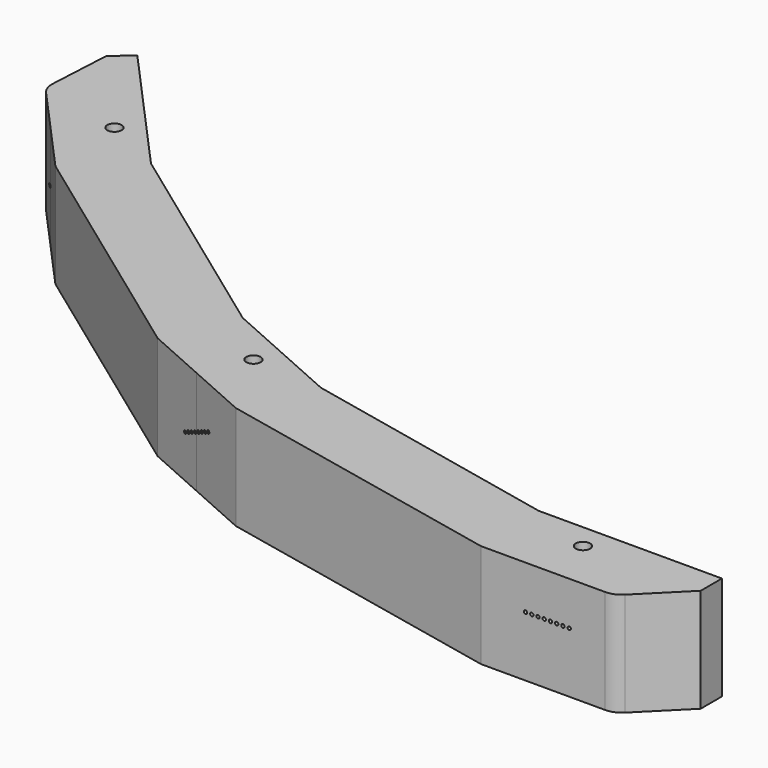
from build123d import *

# Parameters (mm, degrees)
F1_DEPTH        = 25
F2_W            = 17
F2_H            = 14
F3_DEPTH        = 10
F4_W            = 12
F4_H            = 12
F5_DEPTH        = 10
F7_D            = 0.8
F7_CSINK_D      = 0.866
F7_CSINK_ANGLE  = 60
F9_D            = 0.8
F9_CSINK_D      = 0.866
F9_CSINK_ANGLE  = 60
F10_W           = 17
F10_H           = 14
F11_DEPTH       = 10
F13_D           = 0.8
F13_CSINK_D     = 0.866
F13_CSINK_ANGLE = 60
F15_DEPTH       = 1
F17_DEPTH       = 1
F19_DEPTH       = 1
F21_D           = 3.4544
F21_DEPTH       = 14.38125
F21_TIP         = 1.0378064612
F23_D           = 4.2
F23_DEPTH       = 10
F23_TIP         = 1.2618073
F24_R           = 0.5
F25_R           = 0.5
F26_R           = 0.5
F28_D           = 4.2
F28_DEPTH       = 10
F28_TIP         = 1.2618073
F30_D           = 4.2
F30_DEPTH       = 10
F30_TIP         = 1.2618073
F32_D           = 3.02
F32_DEPTH       = 6
F32_TIP         = 0.9072995347
F34_D           = 3.02
F34_DEPTH       = 6
F34_TIP         = 0.9072995347


# Not quite as in the source:
# - a feature names something its author has since deleted; it is built from what else it names


with BuildPart() as f1:
    # F0 (on Top) → F1 (new body)
    with BuildSketch(Plane.XY):
        with BuildLine():
            Line((-195.1064812103, -156.9314377097), (-185.7862063693, -167.2826515897))
            Line((-185.7862063693, -167.2826515897), (-175.0801166676, -179.1729687974))
            Line((-175.0801166676, -179.1729687974), (-116.3008880912, -221.8785781214))
            Line((-116.3008880912, -221.8785781214), (-101.6841607689, -228.3863644107))
            Line((-101.6841607689, -228.3863644107), (-87.0674334467, -234.8941506999))
            Line((-87.0674334467, -234.8941506999), (-16, -250))
            Line((-16, -250), (0, -250))
            Line((0, -250), (13.9289321881, -250))
            ThreePointArc((13.9289321881, -250), (15.84234935, -249.6193976626), (17.4644660941, -248.5355339059))
            Line((17.4644660941, -248.5355339059), (27.610408524, -238.389591476))
            Line((27.610408524, -238.389591476), (27.610408524, -232))
            Line((27.610408524, -232), (-0.4985836237, -232))
            Line((-0.4985836237, -232), (-16.4985836237, -232))
            Line((-16.4985836237, -232), (-79.7461738713, -218.4503324623))
            Line((-79.7461738713, -218.4503324623), (-94.3629011936, -211.9425461731))
            Line((-94.3629011936, -211.9425461731), (-108.9796285159, -205.4347598839))
            Line((-108.9796285159, -205.4347598839), (-161.703509809, -167.1286178829))
            Line((-161.703509809, -167.1286178829), (-172.4095995108, -155.2383006753))
            Line((-172.4095995108, -155.2383006753), (-191.2181864707, -134.3492486113))
            Line((-191.2181864707, -134.3492486113), (-195.596058473, -138.2911022675))
            Line((-195.596058473, -138.2911022675), (-196.3839047567, -153.3241048967))
            ThreePointArc((-196.3839047567, -153.3241048967), (-196.1039645384, -155.2548189741), (-195.1064812103, -156.9314377097))
        make_face()
    extrude(amount=-F1_DEPTH)

    # F2 (on face) → F3 (cut)
    with BuildSketch(Plane(origin=(-94.3629011936, -211.9425461731, 0), x_dir=(-0.9135454576, 0.4067366431, 0), z_dir=(0.4067366431, 0.9135454576, 0))):
        with Locations((0, -12.5)):
            Rectangle(F2_W, F2_H)
    extrude(amount=-F3_DEPTH, mode=Mode.SUBTRACT)

    # F4 (on face) → F5 (cut)
    with BuildSketch(Plane(origin=(-172.4095995108, -155.2383006753, 0), x_dir=(-0.6691306064, 0.7431448255, 0), z_dir=(0.7431448255, 0.6691306064, 0))):
        with Locations((0, -12.5)):
            Rectangle(F4_W, F4_H)
    extrude(amount=-F5_DEPTH, mode=Mode.SUBTRACT)

    # F7 (through all)
    with Locations(Plane(origin=(-179.8410477655, -161.9296067388, 0), x_dir=(-0.6691306064, 0.7431448255, 0), z_dir=(0.7431448255, 0.6691306064, 0))):
        with Locations((4.7581158819, -14.7187458741), (3.3986542014, -14.0848184815), (2.0391925208, -13.4508910889), (0.6797308403, -12.8169636963), (-0.6797308403, -12.1830363037), (-2.0391925208, -11.5491089111), (-3.3986542014, -10.9151815185), (-4.7581158819, -10.2812541259)):
            CounterSinkHole(F7_D / 2, F7_CSINK_D / 2, counter_sink_angle=F7_CSINK_ANGLE)

    # F9 (through all)
    with Locations(Plane(origin=(-98.4302676243, -221.0780007495, 0), x_dir=(-0.9135454576, 0.4067366431, 0), z_dir=(0.4067366431, 0.9135454576, 0))):
        with Locations((4.7581158819, -14.7187458741), (3.3986542014, -14.0848184815), (2.0391925208, -13.4508910889), (0.6797308403, -12.8169636963), (-0.6797308403, -12.1830363037), (-2.0391925208, -11.5491089111), (-3.3986542014, -10.9151815185), (-4.7581158819, -10.2812541259)):
            CounterSinkHole(F9_D / 2, F9_CSINK_D / 2, counter_sink_angle=F9_CSINK_ANGLE)

    # F10 (on face) → F11 (cut)
    with BuildSketch(Plane(origin=(0, -232, 0), x_dir=(-1, 0, 0), z_dir=(0, 1, 0))):
        with Locations((0, -12.5)):
            Rectangle(F10_W, F10_H)
    extrude(amount=-F11_DEPTH, mode=Mode.SUBTRACT)

    # F13 (through all)
    with Locations(Plane(origin=(0, -242, 0), x_dir=(-1, 0, 0), z_dir=(0, 1, 0))):
        with Locations((5.25, -10.5), (3.75, -10.5), (2.25, -10.5), (0.75, -10.5), (-0.75, -10.5), (-2.25, -10.5), (-3.75, -10.5), (-5.25, -10.5)):
            CounterSinkHole(F13_D / 2, F13_CSINK_D / 2, counter_sink_angle=F13_CSINK_ANGLE)

    # F14 (on face) → F15 (cut)
    with BuildSketch(Plane(origin=(-94.3629011936, -211.9425461731, 0), x_dir=(-0.9135454576, 0.4067366431, 0), z_dir=(0.4067366431, 0.9135454576, 0))):
        with BuildLine():
            Line((-9.2, -21.5), (9.2, -21.5))
            ThreePointArc((9.2, -21.5), (9.7656854249, -21.2656854249), (10, -20.7))
            Line((10, -20.7), (10, -4.3))
            ThreePointArc((10, -4.3), (9.7656854249, -3.7343145751), (9.2, -3.5))
            Line((9.2, -3.5), (-9.2, -3.5))
            ThreePointArc((-9.2, -3.5), (-9.7656854249, -3.7343145751), (-10, -4.3))
            Line((-10, -4.3), (-10, -20.7))
            ThreePointArc((-10, -20.7), (-9.7656854249, -21.2656854249), (-9.2, -21.5))
        make_face()
        with BuildLine():
            ThreePointArc((9, -19.7), (8.7656854249, -20.2656854249), (8.2, -20.5))
            Line((8.2, -20.5), (-8.2, -20.5))
            ThreePointArc((-8.2, -20.5), (-8.7656854249, -20.2656854249), (-9, -19.7))
            Line((-9, -19.7), (-9, -5.3))
            ThreePointArc((-9, -5.3), (-8.7656854249, -4.7343145751), (-8.2, -4.5))
            Line((-8.2, -4.5), (8.2, -4.5))
            ThreePointArc((8.2, -4.5), (8.7656854249, -4.7343145751), (9, -5.3))
            Line((9, -5.3), (9, -19.7))
        make_face(mode=Mode.SUBTRACT)
    extrude(amount=-F15_DEPTH, mode=Mode.SUBTRACT)

    # F16 (on face) → F17 (cut)
    with BuildSketch(Plane(origin=(-172.4095995108, -155.2383006753, 0), x_dir=(-0.6691306064, 0.7431448255, 0), z_dir=(0.7431448255, 0.6691306064, 0))):
        with BuildLine():
            Line((-9.2, -21.5), (9.2, -21.5))
            ThreePointArc((9.2, -21.5), (9.7656854249, -21.2656854249), (10, -20.7))
            Line((10, -20.7), (10, -4.3))
            ThreePointArc((10, -4.3), (9.7656854249, -3.7343145751), (9.2, -3.5))
            Line((9.2, -3.5), (-9.2, -3.5))
            ThreePointArc((-9.2, -3.5), (-9.7656854249, -3.7343145751), (-10, -4.3))
            Line((-10, -4.3), (-10, -20.7))
            ThreePointArc((-10, -20.7), (-9.7656854249, -21.2656854249), (-9.2, -21.5))
        make_face()
        with BuildLine():
            ThreePointArc((9, -19.7), (8.7656854249, -20.2656854249), (8.2, -20.5))
            Line((8.2, -20.5), (-8.2, -20.5))
            ThreePointArc((-8.2, -20.5), (-8.7656854249, -20.2656854249), (-9, -19.7))
            Line((-9, -19.7), (-9, -5.3))
            ThreePointArc((-9, -5.3), (-8.7656854249, -4.7343145751), (-8.2, -4.5))
            Line((-8.2, -4.5), (8.2, -4.5))
            ThreePointArc((8.2, -4.5), (8.7656854249, -4.7343145751), (9, -5.3))
            Line((9, -5.3), (9, -19.7))
        make_face(mode=Mode.SUBTRACT)
    extrude(amount=-F17_DEPTH, mode=Mode.SUBTRACT)

    # F18 (on face) → F19 (cut)
    with BuildSketch(Plane(origin=(0, -232, 0), x_dir=(-1, 0, 0), z_dir=(0, 1, 0))):
        with BuildLine():
            Line((-9.2, -21.5), (9.2, -21.5))
            ThreePointArc((9.2, -21.5), (9.7656854249, -21.2656854249), (10, -20.7))
            Line((10, -20.7), (10, -4.3))
            ThreePointArc((10, -4.3), (9.7656854249, -3.7343145751), (9.2, -3.5))
            Line((9.2, -3.5), (-9.2, -3.5))
            ThreePointArc((-9.2, -3.5), (-9.7656854249, -3.7343145751), (-10, -4.3))
            Line((-10, -4.3), (-10, -20.7))
            ThreePointArc((-10, -20.7), (-9.7656854249, -21.2656854249), (-9.2, -21.5))
        make_face()
        with BuildLine():
            ThreePointArc((9, -19.7), (8.7656854249, -20.2656854249), (8.2, -20.5))
            Line((8.2, -20.5), (-8.2, -20.5))
            ThreePointArc((-8.2, -20.5), (-8.7656854249, -20.2656854249), (-9, -19.7))
            Line((-9, -19.7), (-9, -5.3))
            ThreePointArc((-9, -5.3), (-8.7656854249, -4.7343145751), (-8.2, -4.5))
            Line((-8.2, -4.5), (8.2, -4.5))
            ThreePointArc((8.2, -4.5), (8.7656854249, -4.7343145751), (9, -5.3))
            Line((9, -5.3), (9, -19.7))
        make_face(mode=Mode.SUBTRACT)
    extrude(amount=-F19_DEPTH, mode=Mode.SUBTRACT)

    # F21
    with Locations(Plane.XY):
        with Locations((-176.1755610332, -160.0226359772), (-96.803321052, -217.4238189189), (-1.0355339059, -238)):
            Hole(F21_D / 2, depth=F21_DEPTH)
            with Locations((0, 0, -(F21_DEPTH + F21_TIP / 2))):  # 118° drill point
                Cone(0, F21_D / 2, F21_TIP, mode=Mode.SUBTRACT)

    # F23
    with Locations(Plane(origin=(0, -232, 0), x_dir=(-1, 0, 0), z_dir=(0, 1, 0))):
        with Locations((13.2492918119, -4.3), (13.2492918119, -20.7), (-18.560408524, -4.3), (-18.560408524, -20.7)):
            Hole(F23_D / 2, depth=F23_DEPTH)
            with Locations((0, 0, -(F23_DEPTH + F23_TIP / 2))):  # 118° drill point
                Cone(0, F23_D / 2, F23_TIP, mode=Mode.SUBTRACT)

    # F24
    f24_edges = [f1.edges().sort_by_distance(p)[0] for p in [
        (-8.5, -242, -12.5),
        (0, -242, -5.5),
        (8.5, -242, -12.5),
        (0, -242, -19.5),
        (-8.5, -237, -5.5),
        (8.5, -237, -5.5),
        (8.5, -237, -19.5),
    ]]
    fillet(f24_edges, radius=F24_R)

    # F25
    f25_edges = [f1.edges().sort_by_distance(p)[0] for p in [
        (-98.430268, -221.078001, -5.5),
        (-90.665131, -224.535262, -12.5),
        (-88.631448, -219.967535, -5.5),
        (-88.631448, -219.967535, -19.5),
        (-98.430268, -221.078001, -19.5),
        (-106.195404, -217.620739, -12.5),
        (-104.161721, -213.053012, -5.5),
        (-104.161721, -213.053012, -19.5),
    ]]
    fillet(f25_edges, radius=F25_R)

    # F26
    f26_edges = [f1.edges().sort_by_distance(p)[0] for p in [
        (-179.841048, -161.929607, -18.5),
        (-179.841048, -161.929607, -6.5),
        (-175.826264, -166.388476, -12.5),
        (-172.11054, -163.042823, -6.5),
        (-172.11054, -163.042823, -18.5),
        (-183.855831, -157.470738, -12.5),
        (-180.140107, -154.125085, -6.5),
        (-180.140107, -154.125085, -18.5),
    ]]
    fillet(f26_edges, radius=F26_R)

    # F28
    with Locations(Plane(origin=(-94.3629011936, -211.9425461731, 0), x_dir=(-0.9135454576, 0.4067366431, 0), z_dir=(0.4067366431, 0.9135454576, 0))):
        with Locations((-13, -4.3), (-13, -20.7), (13, -4.3), (13, -20.7)):
            Hole(F28_D / 2, depth=F28_DEPTH)
            with Locations((0, 0, -(F28_DEPTH + F28_TIP / 2))):  # 118° drill point
                Cone(0, F28_D / 2, F28_TIP, mode=Mode.SUBTRACT)

    # F30
    with Locations(Plane(origin=(-172.4095995108, -155.2383006753, 0), x_dir=(-0.6691306064, 0.7431448255, 0), z_dir=(0.7431448255, 0.6691306064, 0))):
        with Locations((-13, -4.3), (-13, -20.7), (19.0589921478, -4.3), (19.0589921478, -20.7)):
            Hole(F30_D / 2, depth=F30_DEPTH)
            with Locations((0, 0, -(F30_DEPTH + F30_TIP / 2))):  # 118° drill point
                Cone(0, F30_D / 2, F30_TIP, mode=Mode.SUBTRACT)

    # F32
    with Locations(Plane(origin=(-48.2448517048, -225.1989285856, 0), x_dir=(-0.9778131425, 0.2094790164, 0), z_dir=(0.2094790164, 0.9778131425, 0))):
        with Locations((-23.1390529194, -3.6051168097), (-23.1390529194, -21.3948831903)):
            Hole(F32_D / 2, depth=F32_DEPTH)
            with Locations((0, 0, -(F32_DEPTH + F32_TIP / 2))):  # 118° drill point
                Cone(0, F32_D / 2, F32_TIP, mode=Mode.SUBTRACT)

    # F34
    with Locations(Plane(origin=(-135.3415691624, -186.2816888834, 0), x_dir=(-0.8090169944, 0.5877852523, 0), z_dir=(0.5877852523, 0.8090169944, 0))):
        with Locations((23.2485540845, -3.5816147789), (23.2485540845, -21.4183852211)):
            Hole(F34_D / 2, depth=F34_DEPTH)
            with Locations((0, 0, -(F34_DEPTH + F34_TIP / 2))):  # 118° drill point
                Cone(0, F34_D / 2, F34_TIP, mode=Mode.SUBTRACT)


solid = f1.part
